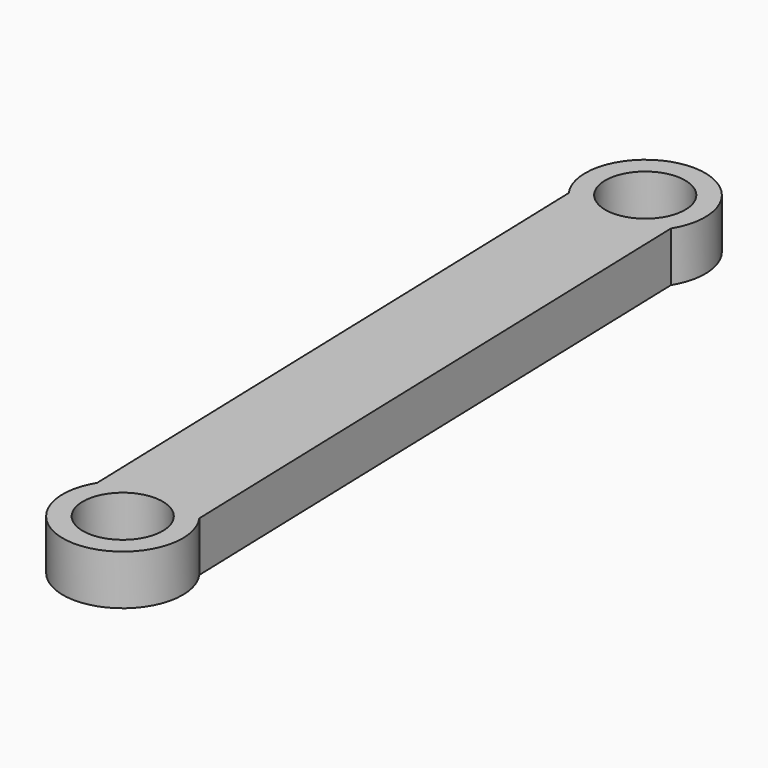
from build123d import *

# Parameters (mm, degrees)
F1_DEPTH = 3.175
F3_D     = 5.08


# Not quite as in the source:
# - a feature names something its author has since deleted; it is built from what else it names


with BuildPart() as f1:
    # F0 (on Top) → F1 (new body)
    with BuildSketch(Plane.XY):
        with BuildLine():
            Line((-3.7668826879, 19.3999561499), (-2.580178634, -19.5931207831))
            ThreePointArc((-2.580178634, -19.5931207831), (0.7733162679, -25.4098573523), (3.7668826879, -19.3999561499))
            Line((3.7668826879, -19.3999561499), (2.580178634, 19.5931207831))
            ThreePointArc((2.580178634, 19.5931207831), (-0.7733162679, 25.4098573523), (-3.7668826879, 19.3999561499))
        make_face()
    extrude(amount=F1_DEPTH)

    # F3 (through all)
    with Locations(Plane.XY.offset(3.175)):
        with Locations((0.6574174881, -21.6016205591), (-0.6574174881, 21.6016205591)):
            Hole(F3_D / 2)


solid = f1.part
